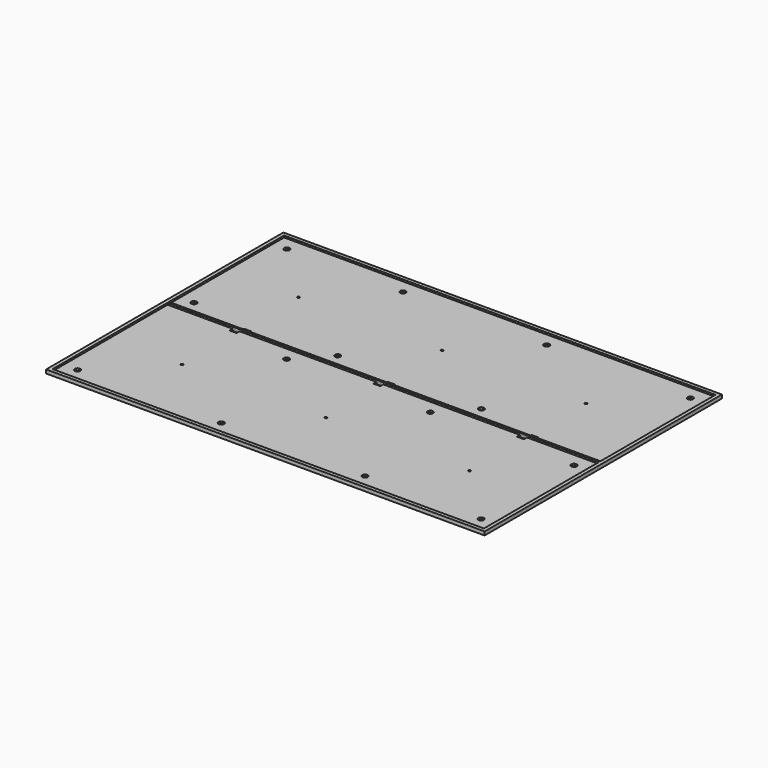
from build123d import *
from build123d import SkipClean  # not in build123d's __all__

# Parameters (mm, degrees)
F0_W     = 244.15
F0_H     = 165.1
F1_DEPTH = 2
F3_DEPTH = 1
F4_R     = 1.55
F4_R_2   = 0.65
F4_W     = 3.9
F4_H     = 2.115
F5_DEPTH = 1.001


with BuildPart() as f1:
    # F0 (on Top) → F1 (new body)
    with BuildSketch(Plane.XY):
        Rectangle(F0_W, F0_H)
    extrude(amount=F1_DEPTH)

    # F2 (on face) → F3 (cut)
    with BuildSketch(Plane.XY.offset(2)):
        Polygon((120.075, 80.55), (-120.075, 80.55), (-120.075, 1), (-120.075, 0.5), (120.075, 0.5), (120.075, 1), align=None)
        Polygon((-120.075, -80.55), (120.075, -80.55), (120.075, -1), (120.075, -0.5), (-120.075, -0.5), (-120.075, -1), align=None)
    extrude(amount=-F3_DEPTH, mode=Mode.SUBTRACT)

    # F4 (on face) → F5 (cut, through all)
    with BuildSketch(Plane.XY.offset(1)):
        with Locations((-47.6721085759, 72.8278914241)):
            Circle(F4_R)
        with Locations((32.3278905301, 72.8278914241)):
            Circle(F4_R)
        with Locations((112.3278914241, 72.8278914241)):
            Circle(F4_R)
        with Locations((-112.3278914241, 8.1721085759)):
            Circle(F4_R)
        with Locations((-32.3278914241, 8.1721085759)):
            Circle(F4_R)
        with Locations((47.6721076818, 8.1721085759)):
            Circle(F4_R)
        with Locations((-80, 40.5)):
            Circle(F4_R_2)
        with Locations((-4.47e-07, 40.5)):
            Circle(F4_R_2)
        with Locations((79.999999553, 40.5)):
            Circle(F4_R_2)
        with Locations((-112.3278914241, -72.8278914241)):
            Circle(F4_R)
        with Locations((-32.3278914241, -72.8278914241)):
            Circle(F4_R)
        with Locations((47.6721076818, -72.8278914241)):
            Circle(F4_R)
        with Locations((112.3278914241, -8.1721085759)):
            Circle(F4_R)
        with Locations((32.3278905301, -8.1721085759)):
            Circle(F4_R)
        with Locations((-47.6721085759, -8.1721085759)):
            Circle(F4_R)
        with Locations((-4.47e-07, -40.5)):
            Circle(F4_R_2)
        with Locations((79.999999553, -40.5)):
            Circle(F4_R_2)
        with Locations((112.3278914241, -72.8278914241)):
            Circle(F4_R)
        with Locations((-112.3278914241, 72.8278914241)):
            Circle(F4_R)
        with Locations((-80, -40.5)):
            Circle(F4_R_2)
        with Locations((-81.949996841, -1.5575)):
            Rectangle(F4_W, F4_H)
        with Locations((-78.0499982119, 1.5575)):
            Rectangle(F4_W, F4_H)
        with Locations((-1.9499991059, -1.5575001072)):
            Rectangle(F4_W, F4_H)
        with Locations((1.9499995232, 1.5575)):
            Rectangle(F4_W, F4_H)
        with Locations((78.0497357585, -1.5575)):
            Rectangle(F4_W, F4_H)
        with Locations((81.9497343876, 1.5575)):
            Rectangle(F4_W, F4_H)
    with SkipClean():  # cleaning this boolean's faces spoils the solid; the shape is the same uncleaned
        extrude(amount=-F5_DEPTH, mode=Mode.SUBTRACT)


solid = f1.part
